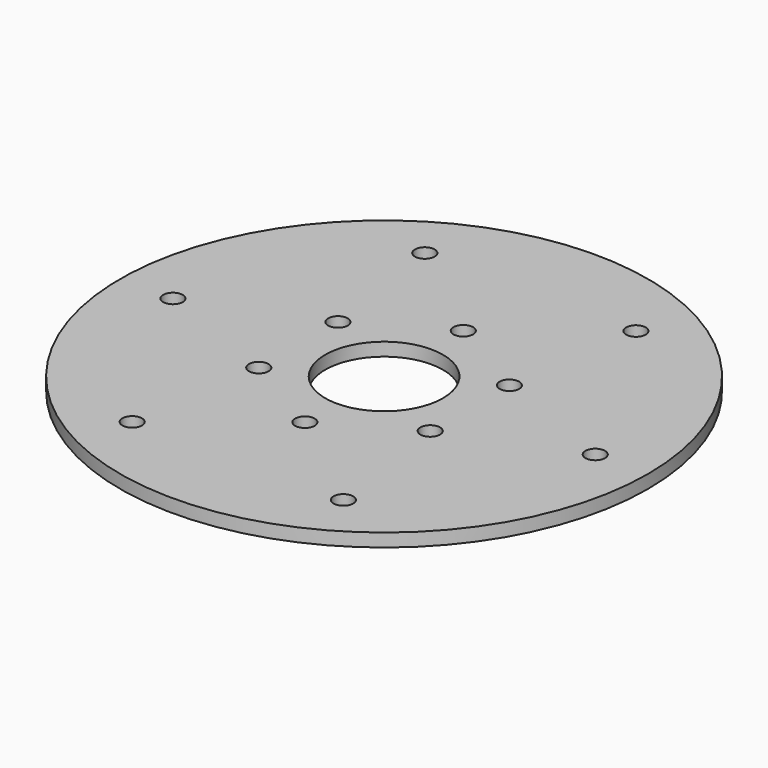
from build123d import *

# Parameters (mm, degrees)
F0_R            = 63.5
F0_R_2          = 14.1605
F1_DEPTH        = 3.175
F2_R            = 2.3622
F3_DEPTH        = 3.176
F3_COPIES_COUNT = 6


# Not quite as in the source:
# - a pattern or mirror of a feature is missing from the dataset's text; its kind, count and spacing are read off the source's solid


with BuildPart() as f1:
    # F0 (on Top) → F1 (new body)
    with BuildSketch(Plane.XY):
        Circle(F0_R)
        Circle(F0_R_2, mode=Mode.SUBTRACT)
    extrude(amount=F1_DEPTH)

    # F2 (on face) → F3 (cut, through all)
    with BuildSketch(Plane.XY.offset(3.175)):
        with Locations((0, 23.8125)):
            Circle(F2_R)
        with Locations((25.4, 43.9940905122)):
            Circle(F2_R)
    f3 = extrude(amount=-F3_DEPTH, mode=Mode.SUBTRACT)

    # F3_copies: F3 ×6 about axis
    f3_copies_axis = Axis((0, 0, 0), (0, 0, 1))
    for i in range(1, F3_COPIES_COUNT):
        add(f3.rotate(f3_copies_axis, i * 360 / F3_COPIES_COUNT), mode=Mode.SUBTRACT)


solid = f1.part
